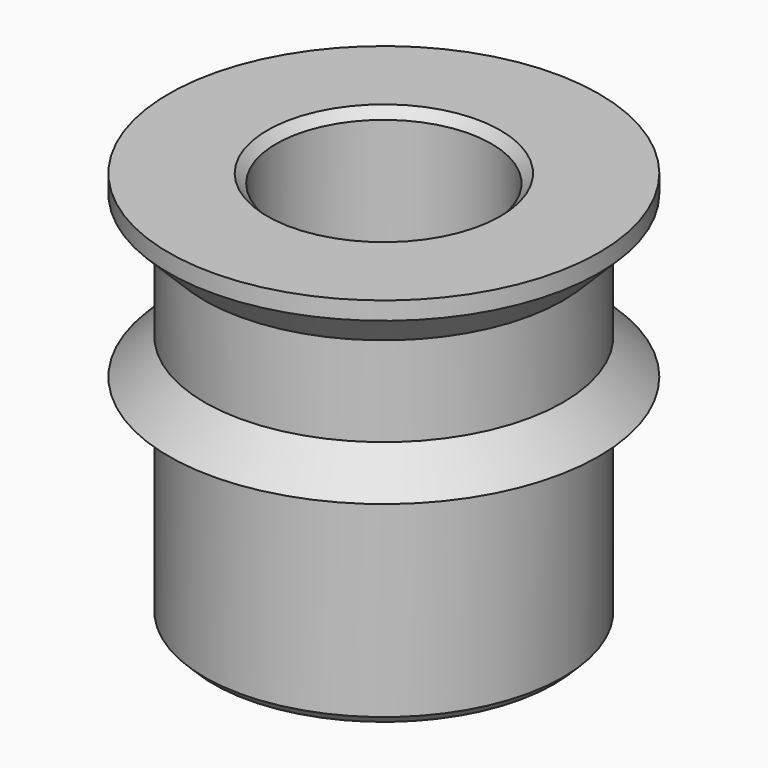
from build123d import *

# Parameters (mm, degrees)
F0_R     = 10
F0_R_2   = 6
F1_DEPTH = 12
F2_R     = 12
F2_R_2   = 6
F3_DEPTH = 2
F4_R     = 10
F4_R_2   = 6
F5_DEPTH = 5
F6_R     = 12
F6_R_2   = 6
F7_DEPTH = 3
F8_SIZE  = 1.99999
F9_SIZE  = 1.99999
F10_SIZE = 0.5


# Not quite as in the source:
# - a fillet or chamfer is up to 0.001 mm smaller than in the source, because OpenCascade refuses the exact size


with BuildPart() as f1:
    # F0 (on Top) → F1 (new body)
    with BuildSketch(Plane.XY):
        Circle(F0_R)
        Circle(F0_R_2, mode=Mode.SUBTRACT)
    extrude(amount=-F1_DEPTH)

    # F2 (on face) → F3 (join)
    with BuildSketch(Plane.XY):
        Circle(F2_R)
        Circle(F2_R_2, mode=Mode.SUBTRACT)
    extrude(amount=F3_DEPTH)

    # F4 (on face) → F5 (join)
    with BuildSketch(Plane.XY.offset(2)):
        Circle(F4_R)
        Circle(F4_R_2, mode=Mode.SUBTRACT)
    extrude(amount=F5_DEPTH)

    # F6 (on face) → F7 (join)
    with BuildSketch(Plane.XY.offset(7)):
        Circle(F6_R)
        Circle(F6_R_2, mode=Mode.SUBTRACT)
    extrude(amount=F7_DEPTH)

    # F8 (size 2 in the source; OpenCascade refuses exactly that, so slightly less here)
    f8_edges = [f1.edges().sort_by_distance(p)[0] for p in [
        (-12, 0, 2),
    ]]
    chamfer(f8_edges, length=F8_SIZE)

    # F9 (size 2 in the source; OpenCascade refuses exactly that, so slightly less here)
    f9_edges = [f1.edges().sort_by_distance(p)[0] for p in [
        (-12, 0, 7),
    ]]
    chamfer(f9_edges, length=F9_SIZE)

    # F10
    f10_edges = [f1.edges().sort_by_distance(p)[0] for p in [
        (-10, 0, -12),
        (-6, 0, -12),
        (-6, 0, 10),
    ]]
    chamfer(f10_edges, length=F10_SIZE)


solid = f1.part
